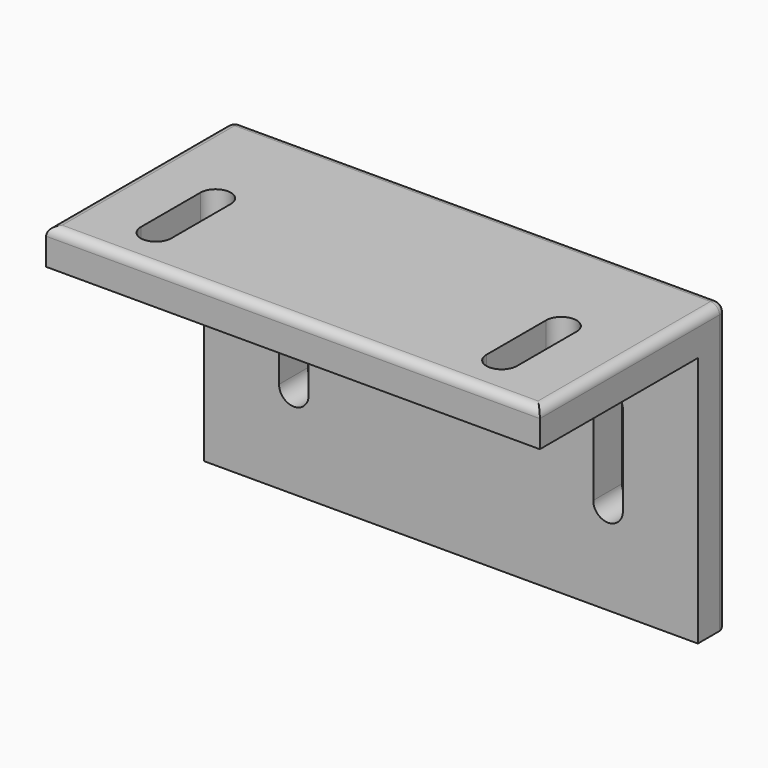
from build123d import *

# Parameters (mm, degrees)
F1_DEPTH = 27.5
F3_DEPTH = 32.001
F4_R     = 1
F6_DEPTH = 26.001


# Not quite as in the source:
# - ends of sketch curves that miss each other by under 0.0002 mm in the source are joined
# - a feature names something its author has since deleted; it is built from what else it names


with BuildPart() as f1:
    # F0 (on Right) → F1 (new body, symmetric)
    with BuildSketch(Plane.YZ):
        Polygon((0, -32), (0, 0), (-26, 0), (-26, -4), (-4, -4), (-4, -32), align=None)
    extrude(amount=F1_DEPTH, both=True)

    # F2 (on Top) → F3 (cut, through all)
    with BuildSketch(Plane.XY):
        with BuildLine():
            Line((-17.55, -21), (-20.95, -21))
            ThreePointArc((-20.95, -21), (-19.25, -22.7), (-17.55, -21))
        make_face()
        with BuildLine():
            Line((-20.95, -12.6989117458), (-20.95, -21))
            Line((-20.95, -21), (-17.55, -21))
            Line((-17.55, -21), (-17.55, -12.6989117458))
            Line((-17.55, -12.6989117458), (-17.55, -12.6936758503))
            ThreePointArc((-17.55, -12.6936758503), (-19.2526179384, -10.9989137616), (-20.95, -12.6989117458))
        make_face()
        with BuildLine():
            ThreePointArc((17.55, -21), (19.25, -22.7), (20.95, -21))
            Line((20.95, -21), (17.55, -21))
        make_face()
        with BuildLine():
            Line((17.55, -21), (20.95, -21))
            Line((20.95, -21), (20.95, -12.6989117458))
            ThreePointArc((20.95, -12.6989117458), (19.2526179384, -10.9989137616), (17.5500080631, -12.6936758752))
            ThreePointArc((17.5500080631, -12.6936758752), (17.5500020158, -12.6962938074), (17.55, -12.6989117458))
            Line((17.55, -12.6989117458), (17.55, -21))
        make_face()
    extrude(amount=-F3_DEPTH, mode=Mode.SUBTRACT)

    # F4
    f4_edges = [f1.edges().sort_by_distance(p)[0] for p in [
        (0, 0, -32),
        (-27.5, 0, -16),
        (27.5, 0, -16),
        (0, 0, 0),
        (0, -26, 0),
        (-27.5, -13, 0),
        (27.5, -13, 0),
    ]]
    fillet(f4_edges, radius=F4_R)

    # F5 (on face) → F6 (cut, through all)
    with BuildSketch(Plane(origin=(0, 0, 0), x_dir=(-1, 0, 0), z_dir=(0, 1, 0))):
        with BuildLine():
            Line((15.85, -11.7517232777), (15.85, -21.7517232777))
            ThreePointArc((15.85, -21.7517232777), (17.5, -23.4017232777), (19.15, -21.7517232777))
            Line((19.15, -21.7517232777), (19.15, -11.7517232777))
            ThreePointArc((19.15, -11.7517232777), (17.5, -10.1017232777), (15.85, -11.7517232777))
        make_face()
        with BuildLine():
            ThreePointArc((-19.15, -21.7517232777), (-17.5, -23.4017232777), (-15.85, -21.7517232777))
            Line((-15.85, -21.7517232777), (-15.85, -11.7517232777))
            ThreePointArc((-15.85, -11.7517232777), (-17.5, -10.1017232777), (-19.15, -11.7517232777))
            Line((-19.15, -11.7517232777), (-19.15, -21.7517232777))
        make_face()
    extrude(amount=-F6_DEPTH, mode=Mode.SUBTRACT)


solid = f1.part
